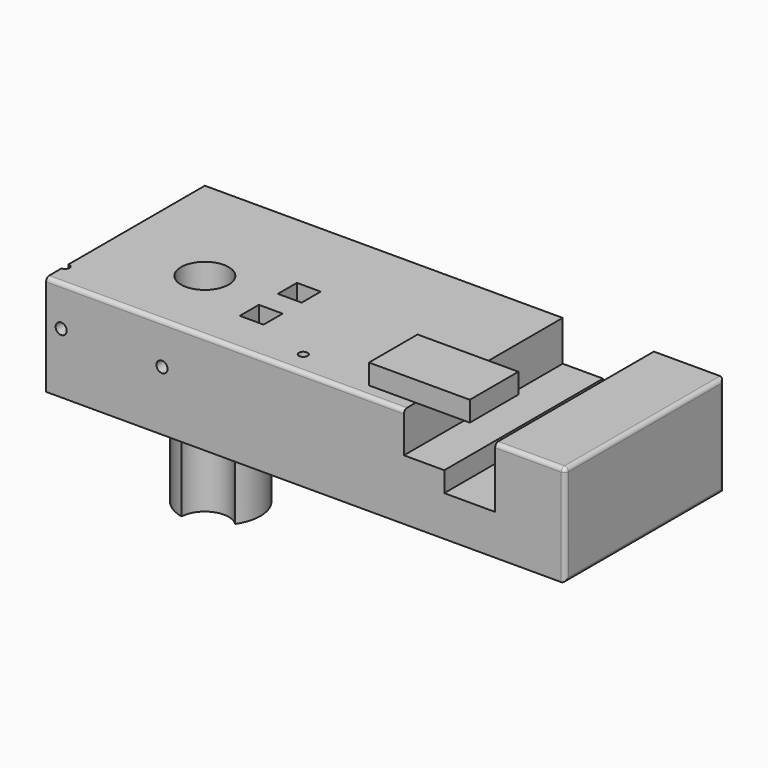
from build123d import *

# Parameters (mm, degrees)
F0_W      = 400
F0_H      = 250
F1_DEPTH  = 127
F2_R      = 50
F3_DEPTH  = 150
F5_D      = 11
F7_D      = 14
F8_DEPTH  = 254
F9_R      = 5.08
F11_DEPTH = 250.001
F12_W     = 127
F12_H     = 76.4771783382
F13_DEPTH = 25.4
F14_W     = 30
F14_H     = 30
F14_R     = 30
F15_DEPTH = 277.001


with BuildPart() as f1:
    # F0 (on Top) → F1 (new body)
    with BuildSketch(Plane.XY):
        with Locations((-200, -125)):
            Rectangle(F0_W, F0_H)
    extrude(amount=F1_DEPTH)

    # F2 (on face) → F3 (join)
    with BuildSketch(Plane(origin=(0, 0, 0), x_dir=(1, 0, 0), z_dir=(0, 0, -1))):
        with Locations((-300, 100)):
            Circle(F2_R)
    extrude(amount=F3_DEPTH)

    # F5 (through all)
    with Locations(Plane(origin=(0, 0, 0), x_dir=(1, 0, 0), z_dir=(0, 0, -1))):
        with Locations((-400, 220), (-100, 220)):
            Hole(F5_D / 2)

    # F7 (through all)
    with Locations(Plane.XZ.offset(250)):
        with Locations((-381, 76.2), (-254, 75.1730280948)):
            Hole(F7_D / 2)

    # F8 (add): a face of the model
    f8_faces = [f1.faces().sort_by_distance(p)[0] for p in [
        (0, -125, 63.5),
    ]]
    extrude(f8_faces, amount=F8_DEPTH)

    # F9
    f9_edges = [f1.edges().sort_by_distance(p)[0] for p in [
        (254, -250, 63.5),
        (254, 0, 63.5),
        (254, -125, 0),
        (254, -125, 127),
        (-73, -250, 127),
    ]]
    fillet(f9_edges, radius=F9_R)

    # F10 (on face) → F11 (cut, through all)
    with BuildSketch(Plane(origin=(0, 0, 0), x_dir=(-1, 0, 0), z_dir=(0, 1, 0))):
        Polygon((-50.8, 127), (-165.6154772818, 127), (-165.6154772818, 50.8), (-101.6, 50.8), (-101.6, 76.2), (-50.8, 76.2), align=None)
    extrude(amount=-F11_DEPTH, mode=Mode.SUBTRACT)

    # F12 (on face) → F13 (join)
    with BuildSketch(Plane.XY.offset(127)):
        with Locations((55.3710968234, -193.1489035487)):
            Rectangle(F12_W, F12_H)
    extrude(amount=F13_DEPTH)

    # F14 (on face) → F15 (cut, through all)
    with BuildSketch(Plane.XY.offset(127)):
        with Locations((-185, -120)):
            Rectangle(F14_W, F14_H)
        with Locations((-185, -180)):
            Rectangle(F14_W, F14_H)
        with Locations((-280, -150)):
            Circle(F14_R)
    extrude(amount=-F15_DEPTH, mode=Mode.SUBTRACT)


solid = f1.part
